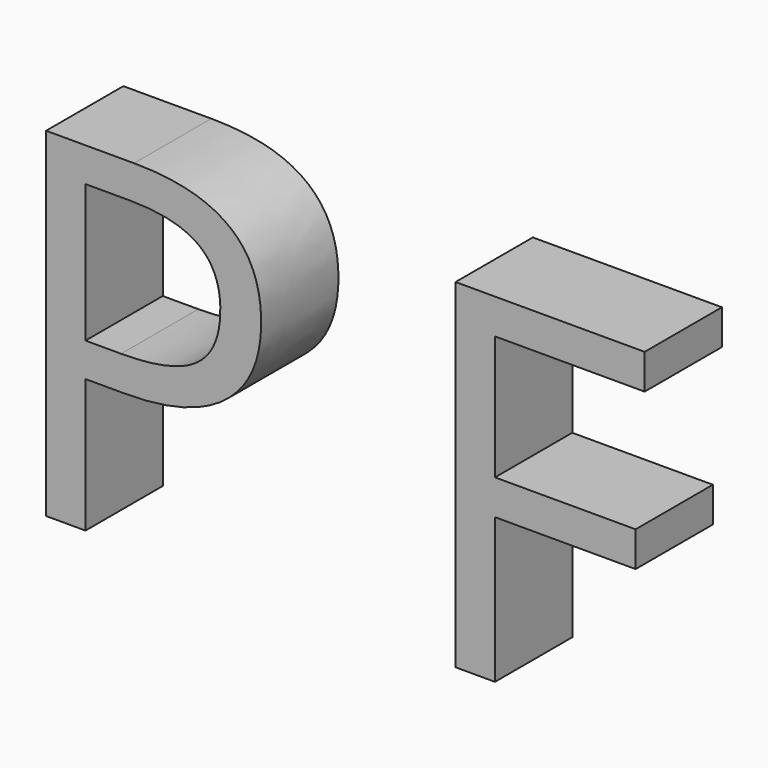
from build123d import *

# Parameters (mm, degrees)
F0_TEXT_SIZE = 124.9637601581
F1_DEPTH     = 25.4


# Not quite as in the source:
# - Text() gives the source's letters only with a copy of the font that has no kerning and outlines rounded to 1/6400 em; it was checked with that copy


with BuildPart() as f1:
    # F0 (on Front) → F1 (new body)
    with BuildSketch(Plane.XZ):
        with Locations((-60.6038895814, -54.6567880534)):
            Text('P F', F0_TEXT_SIZE, font='Open Sans', text_align=(TextAlign.LEFT, TextAlign.BOTTOM))
    extrude(amount=F1_DEPTH)


solid = f1.part
